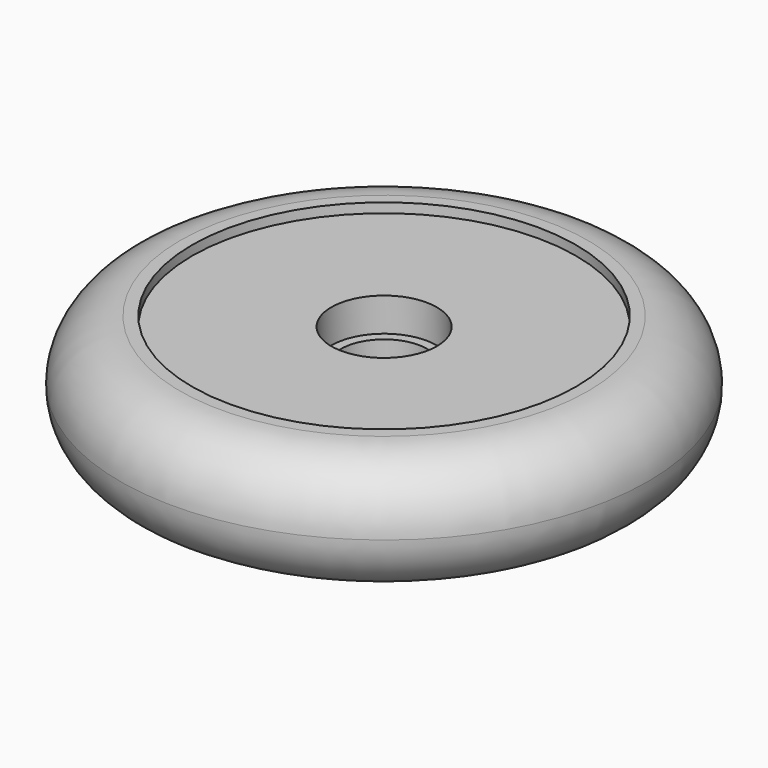
from build123d import *

# Parameters (mm, degrees)
F0_R      = 55
F1_DEPTH  = 25
F2_R      = 40
F3_DEPTH  = 2
F4_R      = 11
F5_DEPTH  = 7
F6_R      = 40
F7_DEPTH  = 2
F8_R      = 11
F9_DEPTH  = 7
F10_R     = 9
F11_DEPTH = 25
F12_R     = 12.49999


# Not quite as in the source:
# - a fillet or chamfer is up to 0.001 mm smaller than in the source, because OpenCascade refuses the exact size


with BuildPart() as f1:
    # F0 (on Top) → F1 (new body)
    with BuildSketch(Plane.XY):
        Circle(F0_R)
    extrude(amount=F1_DEPTH)

    # F2 (on face) → F3 (cut)
    with BuildSketch(Plane.XY.offset(25)):
        Circle(F2_R)
    extrude(amount=-F3_DEPTH, mode=Mode.SUBTRACT)

    # F4 (on face) → F5 (cut)
    with BuildSketch(Plane.XY.offset(23)):
        Circle(F4_R)
    extrude(amount=-F5_DEPTH, mode=Mode.SUBTRACT)

    # F6 (on face) → F7 (cut)
    with BuildSketch(Plane(origin=(0, 0, 0), x_dir=(1, 0, 0), z_dir=(0, 0, -1))):
        Circle(F6_R)
    extrude(amount=-F7_DEPTH, mode=Mode.SUBTRACT)

    # F8 (on face) → F9 (cut)
    with BuildSketch(Plane(origin=(0, 0, 2), x_dir=(1, 0, 0), z_dir=(0, 0, -1))):
        Circle(F8_R)
    extrude(amount=-F9_DEPTH, mode=Mode.SUBTRACT)

    # F10 (on face) → F11 (cut)
    with BuildSketch(Plane.XY.offset(16)):
        Circle(F10_R)
    extrude(amount=-F11_DEPTH, mode=Mode.SUBTRACT)

    # F12 (radius 12.5 in the source; OpenCascade refuses exactly that, so slightly less here)
    f12_edges = [f1.edges().sort_by_distance(p)[0] for p in [
        (-55, 0, 25),
        (-55, 0, 0),
    ]]
    fillet(f12_edges, radius=F12_R)


solid = f1.part
